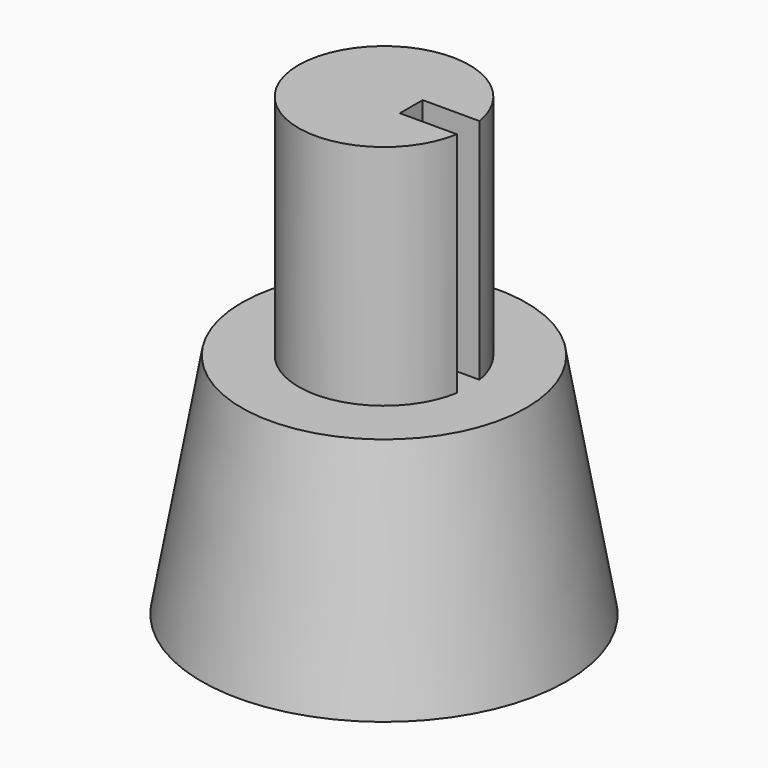
from build123d import *

# Parameters (mm, degrees)
F3_DEPTH = 50.8
F4_R     = 31.75
F5_DEPTH = 50.8
F5_TAPER = -10


# Not quite as in the source:
# - the program builds the solid bodies; features that only make, move or delete a surface that nothing else refers to are left out


with BuildPart() as f3:
    # F2 (on face) → F3 (new body)
    with BuildSketch(Plane.XY.offset(-76.2)):
        with BuildLine():
            Line((6.0835533113, 3.175), (18.7835533113, 3.175))
            ThreePointArc((18.7835533113, 3.175), (-19.05, 0), (18.7835533113, -3.175))
            Line((18.7835533113, -3.175), (6.0835533113, -3.175))
            Line((6.0835533113, -3.175), (6.0835533113, 3.175))
        make_face()
    extrude(amount=-F3_DEPTH)

    # F4 (on face) → F5 (join)
    with BuildSketch(Plane(origin=(0, 0, -127), x_dir=(1, 0, 0), z_dir=(0, 0, -1))):
        Circle(F4_R)
    extrude(amount=F5_DEPTH, taper=F5_TAPER)


solid = f3.part
